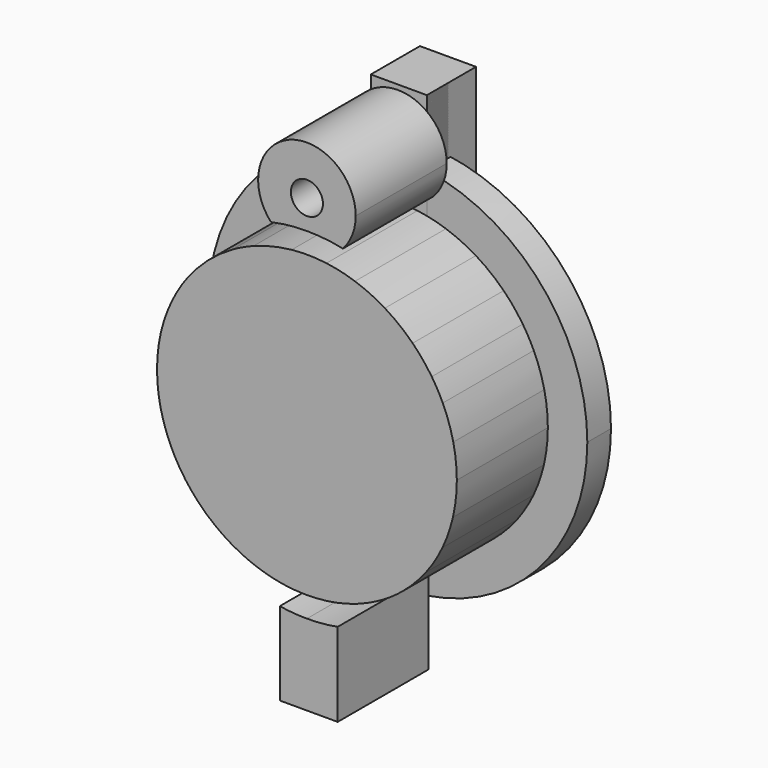
from build123d import *

# Parameters (mm, degrees)
F1_DEPTH = 25.4
F0_R     = 3.5759334616
F2_W     = 10.2924144245
F2_H     = 26.7821848836
F3_DEPTH = 6.604
F4_W     = 12.5268190168
F4_H     = 5.8593181893
F5_DEPTH = 56.388
F7_DEPTH = 13.716


# Not quite as in the source:
# - a feature names something its author has since deleted; it is built from what else it names


with BuildPart() as f1:
    # F0 (on Front) → F1 (new body)
    with BuildSketch(Plane.XZ):
        with BuildLine():
            Line((6.8695456721, -56.1686381698), (6.8695456721, -37.4755832811))
            ThreePointArc((6.8695456721, -37.4755832811), (3.4489329502, -37.9435747065), (0, -38.1))
            ThreePointArc((0, -38.1), (-3.0403780557, -37.9784952477), (-6.0613639653, -37.6147559726))
            Line((-6.0613639653, -37.6147559726), (-6.0613639653, -56.1686381698))
            Line((-6.0613639653, -56.1686381698), (6.8695456721, -56.1686381698))
        make_face()
    extrude(amount=F1_DEPTH)

    # F2 (on Front) → F3 (join)
    with BuildSketch(Plane.XZ):
        with BuildLine():
            ThreePointArc((5.4433241836, 41.9355938654), (-31.7679698214, -27.910928047), (42.2873954154, 0))
            ThreePointArc((42.2873954154, 0), (31.7679698214, 27.910928047), (5.4433241836, 41.9355938654))
        make_face()
        with Locations((0.2971169714, 28.5445014237)):
            Rectangle(F2_W, F2_H, mode=Mode.SUBTRACT)
        with Locations((0.2971169714, 28.5445014237)):
            Rectangle(F2_W, F2_H)
    extrude(amount=-F3_DEPTH)

    # F4 (on Top) → F5 (join)
    with BuildSketch(Plane.XY):
        with Locations((0.2020455431, 2.9296590947)):
            Rectangle(F4_W, F4_H)
    extrude(amount=F5_DEPTH)


with BuildPart() as f1b:
    # F0 (on Front) → F1, piece 2 (new body)
    with BuildSketch(Plane.XZ):
        with BuildLine():
            ThreePointArc((4.487961354, -33.1679662969), (5.6824578, -32.9843214079), (6.8695456721, -32.7576728057))
            Line((6.8695456721, -32.7576728057), (6.8695456721, 0))
            Line((6.8695456721, 0), (-6.0613639653, 0))
            Line((-6.0613639653, 0), (-6.0613639653, -32.9167989371))
            ThreePointArc((-6.0613639653, -32.9167989371), (-4.4704378889, -33.1703326855), (-2.8691550351, -33.3470198784))
            ThreePointArc((-2.8691550351, -33.3470198784), (0.8143393155, -33.460314357), (4.487961354, -33.1679662969))
        make_face()
        with BuildLine():
            ThreePointArc((33.4702223684, 0), (33.272080661, 3.6365414714), (32.6800015131, 7.2300267283))
            ThreePointArc((32.6800015131, 7.2300267283), (31.6959035362, 10.7529291085), (30.3332592567, 14.147408535))
            ThreePointArc((30.3332592567, 14.147408535), (29.1850865539, 16.3855579164), (27.872065839, 18.5311556913))
            ThreePointArc((27.872065839, 18.5311556913), (25.8717499893, 21.2346023716), (23.6102379161, 23.7236685809))
            ThreePointArc((23.6102379161, 23.7236685809), (20.6514709993, 26.3395620873), (17.4051758786, 28.588732711))
            ThreePointArc((17.4051758786, 28.588732711), (14.1530883003, 30.3306095711), (10.7290520592, 31.7039938698))
            ThreePointArc((10.7290520592, 31.7039938698), (7.5814317421, 32.6002711358), (4.361324943, 33.1848554333))
            ThreePointArc((4.361324943, 33.1848554333), (0.487779565, 33.4666678425), (-3.3923335593, 33.2978656735))
            ThreePointArc((-3.3923335593, 33.2978656735), (-7.7171351235, 32.5684143132), (-11.9094251007, 31.2797279265))
            ThreePointArc((-11.9094251007, 31.2797279265), (-14.2871844632, 30.2676749272), (-16.5797760555, 29.0751923697))
            ThreePointArc((-16.5797760555, 29.0751923697), (-20.8481995979, 26.1841241769), (-24.6220061868, 22.6718459046))
            ThreePointArc((-24.6220061868, 22.6718459046), (-26.2829079823, 20.7235260847), (-27.7900301655, 18.65395424))
            ThreePointArc((-27.7900301655, 18.65395424), (-29.6857638641, 15.4599873607), (-31.2159364419, 12.0756406638))
            ThreePointArc((-31.2159364419, 12.0756406638), (-32.329615965, 8.6632394024), (-33.0714522967, 5.1511967907))
            ThreePointArc((-33.0714522967, 5.1511967907), (-33.4448970679, 1.3017855076), (-33.3717923511, -2.5650069518))
            ThreePointArc((-33.3717923511, -2.5650069518), (-32.9310119846, -5.9836640162), (-32.1409632297, -9.338857963))
            ThreePointArc((-32.1409632297, -9.338857963), (-30.9869503626, -12.6516675823), (-29.4925335792, -15.8254936248))
            ThreePointArc((-29.4925335792, -15.8254936248), (-27.7649468656, -18.6912683074), (-25.7598429697, -21.3702193616))
            ThreePointArc((-25.7598429697, -21.3702193616), (-23.3143984723, -24.0144666662), (-20.5989798878, -26.3806332935))
            ThreePointArc((-20.5989798878, -26.3806332935), (-17.7174099154, -28.3962879841), (-14.6402605275, -30.0984809762))
            ThreePointArc((-14.6402605275, -30.0984809762), (-12.3713467967, -31.0999286788), (-10.0345070529, -31.9306193738))
            ThreePointArc((-10.0345070529, -31.9306193738), (-8.0630269435, -32.4845098762), (-6.0613639653, -32.9167989371))
            Line((-6.0613639653, -32.9167989371), (-6.0613639653, 0))
            Line((-6.0613639653, 0), (6.8695456721, 0))
            Line((6.8695456721, 0), (6.8695456721, -32.7576728057))
            ThreePointArc((6.8695456721, -32.7576728057), (9.1234535866, -32.2027697573), (11.3334810452, -31.492983231))
            ThreePointArc((11.3334810452, -31.492983231), (14.4425159933, -30.1938655553), (17.4051758786, -28.588732711))
            ThreePointArc((17.4051758786, -28.588732711), (19.4071458434, -27.2693688156), (21.3095278268, -25.8100718555))
            ThreePointArc((21.3095278268, -25.8100718555), (24.1105991279, -23.2149692026), (26.5978617447, -20.3177148321))
            ThreePointArc((26.5978617447, -20.3177148321), (28.5872814702, -17.407559379), (30.2595876325, -14.3043050057))
            ThreePointArc((30.2595876325, -14.3043050057), (31.6117063333, -10.9979910932), (32.6037613985, -7.5664078701))
            ThreePointArc((32.6037613985, -7.5664078701), (33.2529015985, -3.8079286584), (33.4702223684, 0))
        make_face()
    extrude(amount=F1_DEPTH)


with BuildPart() as f1c:
    # F0 (on Front) → F1, piece 3 (new body)
    with BuildSketch(Plane.XZ):
        with BuildLine():
            ThreePointArc((0, 38.1), (4.0384296709, 37.8853677004), (8.0313592133, 37.243889018))
            ThreePointArc((8.0313592133, 37.243889018), (10.151987984, 40.6546224187), (10.8924189561, 44.6020178497))
            ThreePointArc((10.8924189561, 44.6020178497), (-3.947395431, 54.7540058337), (-8.0313592133, 37.243889018))
            ThreePointArc((-8.0313592133, 37.243889018), (-4.0384296709, 37.8853677004), (0, 38.1))
        make_face()
        with Locations((0, 44.6020178497)):
            Circle(F0_R, mode=Mode.SUBTRACT)
    extrude(amount=F1_DEPTH)


with BuildPart() as f7:
    # F6 (on Front) → F7 (new body)
    with BuildSketch(Plane.XZ):
        with BuildLine():
            ThreePointArc((6.4654545859, -3.9437694851), (7.2911069745, -2.0482138168), (7.5733361706, 0))
            ThreePointArc((7.5733361706, 0), (7.2911069745, 2.0482138168), (6.4654545859, 3.9437694851))
            Line((6.4654545859, 3.9437694851), (6.4654545859, -3.9437694851))
        make_face()
        with BuildLine():
            Line((6.4654545859, -3.9437694851), (6.4654545859, 3.9437694851))
            ThreePointArc((6.4654545859, 3.9437694851), (0.3602992694, 7.564760749), (-6.0613648966, 4.5404048656))
            Line((-6.0613648966, 4.5404048656), (-6.0613648966, -4.5404048656))
            ThreePointArc((-6.0613648966, -4.5404048656), (0.3602992694, -7.564760749), (6.4654545859, -3.9437694851))
        make_face()
        with BuildLine():
            ThreePointArc((-6.0613648966, 4.5404048656), (0.3602992694, 7.564760749), (6.4654545859, 3.9437694851))
            Line((6.4654545859, 3.9437694851), (6.4654545859, 56.572727859))
            Line((6.4654545859, 56.572727859), (-6.0613648966, 56.572727859))
            Line((-6.0613648966, 56.572727859), (-6.0613648966, 4.5404048656))
        make_face()
        with BuildLine():
            Line((6.4654545859, -17.7800003439), (6.4654545859, -3.9437694851))
            ThreePointArc((6.4654545859, -3.9437694851), (0.3602992694, -7.564760749), (-6.0613648966, -4.5404048656))
            Line((-6.0613648966, -4.5404048656), (-6.0613648966, -17.7800003439))
            Line((-6.0613648966, -17.7800003439), (6.4654545859, -17.7800003439))
        make_face()
        with BuildLine():
            Line((-6.0613648966, -4.5404048656), (-6.0613648966, 4.5404048656))
            ThreePointArc((-6.0613648966, 4.5404048656), (-7.5733361706, 0), (-6.0613648966, -4.5404048656))
        make_face()
    extrude(amount=-F7_DEPTH)


solid = Compound([f1.part, f1b.part, f1c.part, f7.part])
